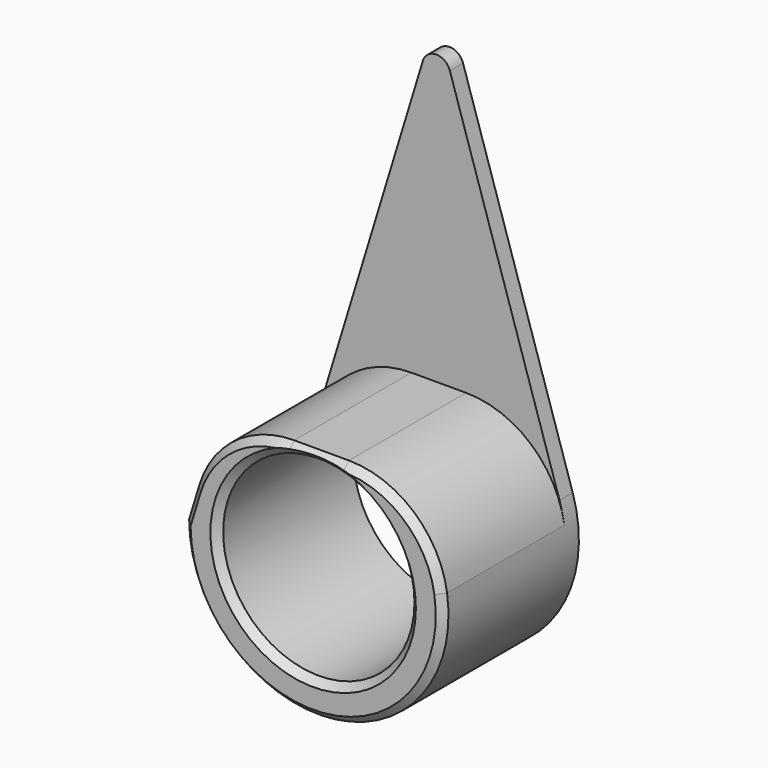
from build123d import *

# Parameters (mm, degrees)
F0_R          = 3.375
F1_DEPTH      = 6
F2_W          = 8.3882776671
F2_H          = 17.9039358627
F3_DEPTH      = 4.576
F3_DEPTH_BACK = 25
F4_T1_DEPTH   = 13.2089304981
F4_T3_DEPTH   = 11.8980683562
F5_R          = 0.5
F6_T1_DEPTH   = 1.9309283779
F6_T3_DEPTH   = 2.3257264643
F6_T8_ANGLE   = 73.0382941175
F6_T10_ANGLE  = 81.5443380081
F6_T12_ANGLE  = 196.5215831172


# Not quite as in the source:
# - a fillet or chamfer that OpenCascade refuses, or shapes differently, is made with other operations: its cross-section is extruded or revolved along the edge and cut away or added


with BuildPart() as f1:
    # F0 (on Front) → F1 (new body)
    with BuildSketch(Plane.XZ):
        with BuildLine():
            Line((0, 15), (-4.575, 0))
            ThreePointArc((-4.575, 0), (0.7061497994, -4.5201744945), (4.3570120047, 1.395375))
            Line((4.3570120047, 1.395375), (0, 15))
        make_face()
        Circle(F0_R, mode=Mode.SUBTRACT)
    extrude(amount=F1_DEPTH)

    # F2 (on Right) → F3 (cut, two sides)
    with BuildSketch(Plane.YZ) as f3_sk:
        with Locations((-4.7752561222, 12.6100402558)):
            Rectangle(F2_W, F2_H)
    extrude(amount=-F3_DEPTH, mode=Mode.SUBTRACT)
    extrude(f3_sk.sketch, amount=F3_DEPTH_BACK, mode=Mode.SUBTRACT)

    # F4: fillet of radius 3.5 on 2 edges, made by hand

    # F4_s2 → F4_t1 (cut)
    with BuildSketch(Plane.XZ.offset(0.5811172887)):
        with BuildLine():
            ThreePointArc((4.5252695152, 0.6727264041), (3.3489995726, 2.8086655863), (1.0633146948, 3.6580723245))
            Line((1.0633146948, 3.6580723245), (1.0633146948, 4.0080723245))
            Line((1.0633146948, 4.0080723245), (3.6323614241, 4.0080723245))
            Line((3.6323614241, 4.0080723245), (3.9656847468, 3.7648223245))
            ThreePointArc((3.9656847468, 3.7648223245), (4.6903353275, 1.502125), (4.8714649972, 0.7241918121))
            Line((4.8714649972, 0.7241918121), (4.5252695152, 0.6727264041))
        make_face()
    extrude(amount=F4_T1_DEPTH, mode=Mode.SUBTRACT)

    # F4_s4 → F4_t3 (cut)
    with BuildSketch(Plane.XZ.offset(0.5811172887)):
        with BuildLine():
            ThreePointArc((-4.2153635131, 1.1791360226), (-2.9504335333, 2.9708754587), (-0.8676136831, 3.6580723245))
            Line((-0.8676136831, 3.6580723245), (-3.459287941, 3.6580723245))
            Line((-3.459287941, 3.6580723245), (-4.2153635131, 1.1791360226))
        make_face()
    extrude(amount=F4_T3_DEPTH, mode=Mode.SUBTRACT)

    # F5
    f5_edges = [f1.edges().sort_by_distance(p)[0] for p in [
        (0, -0.290559, 15),
    ]]
    fillet(f5_edges, radius=F5_R)

    # F6: chamfer of 0.25 on 6 edges, made by hand

    # F6_s2 → F6_t1 (cut)
    with BuildSketch(Plane.YZ.offset(-0.8676136831)):
        Polygon((-6, 3.4080723245), (-5.75, 3.6580723245), (-6, 3.6580723245), align=None)
    extrude(amount=F6_T1_DEPTH, mode=Mode.SUBTRACT)

    # F6_s4 → F6_t3 (cut)
    with BuildSketch(Plane(origin=(-0.0297318944, 0, -0.0974816211), x_dir=(0, 1, 0), z_dir=(-0.2917324852, 0, -0.9564999514))):
        Polygon((-5.75, -4.3759872778), (-6, -4.1259872778), (-6, -4.3759872778), align=None)
    extrude(amount=F6_T3_DEPTH, mode=Mode.SUBTRACT)

    # F6_s5 → F6_t6 (revolve, cut)
    with BuildSketch(Plane.XY):
        Polygon((3.375, -5.75), (3.625, -6), (3.375, -6), align=None)
    revolve(axis=Axis((0, -6, 0), (0, -1, 0)), mode=Mode.SUBTRACT)

    # F6_s7 → F6_t8 (revolve, cut)
    with BuildSketch(Plane(origin=(-0.0297318944, 0, -0.0974816209), x_dir=(0, 1, 0), z_dir=(-0.2917324851, 0, -0.9564999514))):
        Polygon((-6, -4.1259872778), (-5.75, -4.3759872778), (-6, -4.3759872778), align=None)
    revolve(axis=Axis((-0.8676136832, -6, 0.1580723246), (0, 1, 0)), revolution_arc=F6_T8_ANGLE, mode=Mode.SUBTRACT)

    # F6_s9 → F6_t10 (revolve, cut)
    with BuildSketch(Plane.YZ.offset(1.0633146948)):
        Polygon((-5.75, 3.6580723245), (-6, 3.4080723245), (-6, 3.6580723245), align=None)
    revolve(axis=Axis((1.0633146948, -6, 0.1580723245), (0, 1, 0)), revolution_arc=F6_T10_ANGLE, mode=Mode.SUBTRACT)

    # F6_s11 → F6_t12 (revolve, cut)
    with BuildSketch(Plane(origin=(0, 0, 0), x_dir=(0, 1, 0), z_dir=(0.1403123523, 0, 0.990107289))):
        Polygon((-5.75, 4.575), (-6, 4.325), (-6, 4.575), align=None)
    revolve(axis=Axis((0, -6, 0), (0, -1, 0)), revolution_arc=F6_T12_ANGLE, mode=Mode.SUBTRACT)


solid = f1.part
